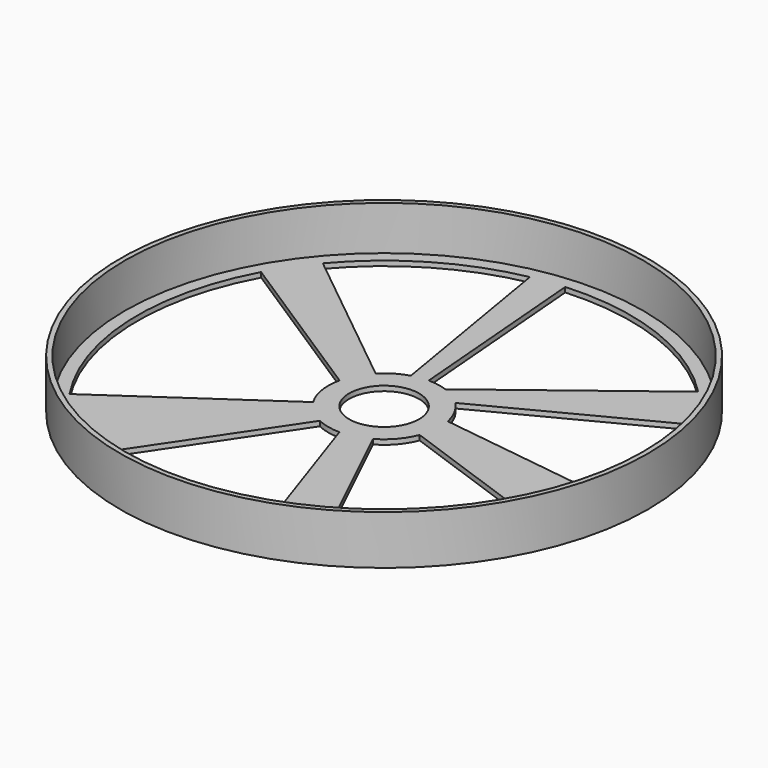
from build123d import *

# Parameters (mm, degrees)
F4_R      = 53.6942028964
F5_DEPTH  = 10
F6_T      = -1
F11_R     = 7.1329818057
F12_DEPTH = 62.1
F13_R     = 7.1161383354
F14_DEPTH = 79.5
F16_DEPTH = 25


# Not quite as in the source:
# - the program builds the solid bodies; features that only make, move or delete a surface that nothing else refers to are left out


with BuildPart() as f5:
    # F4 (on Top) → F5 (new body)
    with BuildSketch(Plane.XY):
        Circle(F4_R)
    extrude(amount=F5_DEPTH)

    # F6
    f6_openings = [f5.faces().sort_by_distance(p)[0] for p in [
        (0, 0, 10),
    ]]
    offset(amount=F6_T, openings=f6_openings)

    # F11 (on Top) → F12 (cut)
    with BuildSketch(Plane.XY):
        Circle(F11_R)
    extrude(amount=-F12_DEPTH, mode=Mode.SUBTRACT)

    # F13 (on Top) → F14 (cut)
    with BuildSketch(Plane.XY):
        Circle(F13_R)
    extrude(amount=F14_DEPTH, mode=Mode.SUBTRACT)

    # F15 (on face) → F16 (cut)
    with BuildSketch(Plane(origin=(0, 0, 0), x_dir=(1, 0, 0), z_dir=(0, 0, -1))):
        with BuildLine():
            Line((0, 11.3609913542), (12.56390222, 48.5457946048))
            ThreePointArc((12.56390222, 48.5457946048), (-7.6213284004, 49.5626993435), (-26.5685055521, 42.5283473172))
            Line((-26.5685055521, 42.5283473172), (-4.8620371636, 10.2680435901))
            ThreePointArc((-4.8620371636, 10.2680435901), (-2.4916831758, 11.0843871955), (0, 11.3609913542))
        make_face()
        with BuildLine():
            Line((-9.7046168543, 5.9069904572), (-41.6567469595, 27.9152511283))
            ThreePointArc((-41.6567469595, 27.9152511283), (-50.0893104585, 2.3678662526), (-44.1043633563, -23.8610759552))
            Line((-44.1043633563, -23.8610759552), (-11.0760480746, -2.5284943342))
            ThreePointArc((-11.0760480746, -2.5284943342), (-11.2137576056, 1.8231195549), (-9.7046168543, 5.9069904572))
        make_face()
        with BuildLine():
            ThreePointArc((-38.3285737992, -32.3336704276), (-25.4491957444, -43.2074559395), (-9.6943225855, -49.1992471732))
            Line((-9.6943225855, -49.1992471732), (-3.2570755528, -10.8840977298))
            ThreePointArc((-3.2570755528, -10.8840977298), (-5.8587236117, -9.733831835), (-8.0930813532, -7.9733405019))
            Line((-8.0930813532, -7.9733405019), (-38.3285737992, -32.3336704276))
        make_face()
        with BuildLine():
            ThreePointArc((-3.1826565415, -50.0441456131), (17.9564047347, -46.8200100577), (35.8302023129, -35.0819385869))
            Line((35.8302023129, -35.0819385869), (3.9370343752, -10.6570110668))
            ThreePointArc((3.9370343752, -10.6570110668), (1.9997392278, -11.183611562), (0, -11.3609913542))
            Line((0, -11.3609913542), (-3.1826565415, -50.0441456131))
        make_face()
        with BuildLine():
            ThreePointArc((42.8675483184, -26.0176692648), (48.2915604345, -13.5081828387), (50.1452471606, 0))
            ThreePointArc((50.1452471606, 0), (50.1236727364, 1.4707971358), (50.058968028, 2.9403286841))
            Line((50.058968028, 2.9403286841), (11.1284959107, -2.2866358071))
            ThreePointArc((11.1284959107, -2.2866358071), (10.0225700646, -5.3497863368), (8.0930813532, -7.9733405019))
            Line((8.0930813532, -7.9733405019), (42.8675483184, -26.0176692648))
        make_face()
        with BuildLine():
            Line((10.5704846038, 4.1637699011), (47.1017248223, 17.2038754811))
            ThreePointArc((47.1017248223, 17.2038754811), (37.4128970239, 33.3889345305), (22.4298275607, 44.8491766747))
            Line((22.4298275607, 44.8491766747), (5.6516858546, 9.8554843387))
            ThreePointArc((5.6516858546, 9.8554843387), (8.5958482365, 7.4285609403), (10.5704846038, 4.1637699011))
        make_face()
    extrude(amount=-F16_DEPTH, mode=Mode.SUBTRACT)


solid = f5.part
